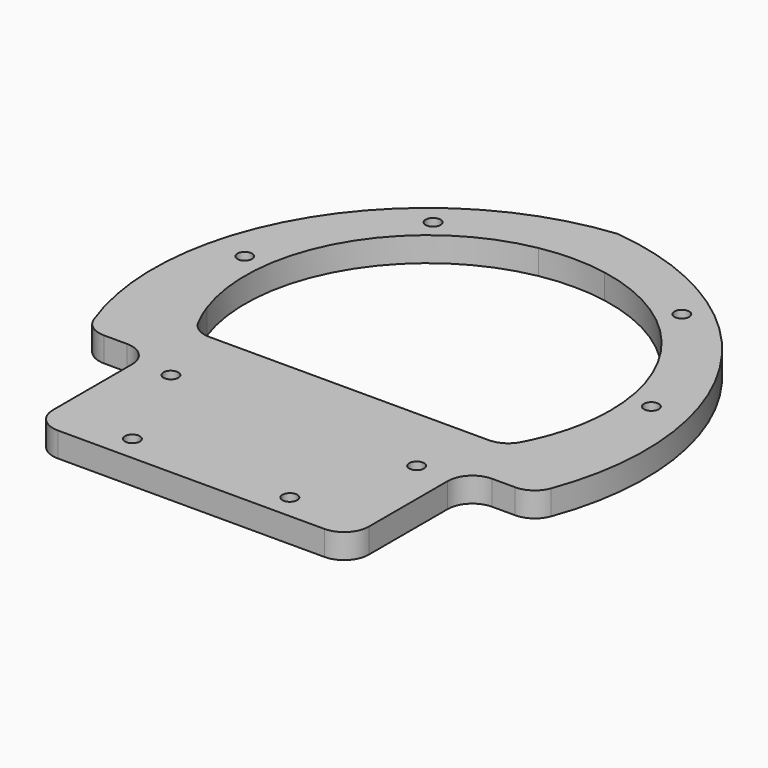
from build123d import *

# Parameters (mm, degrees)
F0_R     = 1.5
F1_DEPTH = 5
F2_R     = 5


# Not quite as in the source:
# - a feature names something its author has since deleted; it is built from what else it names


with BuildPart() as f1:
    # F0 (on Top) → F1 (new body)
    with BuildSketch(Plane.XY):
        with BuildLine():
            Line((32, -25.9806431703), (45.0002060157, -25.9806431703))
            Line((45.0002060157, -25.9806431703), (34.8648160141, -8.425632733))
            ThreePointArc((34.8648160141, -8.425632733), (33.2306953855, -12.3086021935), (31.1657699329, -15.9806431703))
            Line((31.1657699329, -15.9806431703), (32, -15.9806431703))
            Line((32, -15.9806431703), (32, -25.9806431703))
        make_face()
        with BuildLine():
            Line((34.8648160141, -8.425632733), (45.0002060157, -25.9806431703))
            ThreePointArc((45.0002060157, -25.9806431703), (42.4187903028, 24.4905), (0.0002060157, 51.9616431703))
            Line((0.0002060157, 51.9616431703), (6.7047123911, 40.3490974884))
            ThreePointArc((6.7047123911, 40.3490974884), (28.4347881869, 27.6357391565), (37, 3.9616431703))
            ThreePointArc((37, 3.9616431703), (36.4622969142, -2.3233312719), (34.8648160141, -8.425632733))
        make_face()
        with Locations((41.2026322213, 9.0961922878)):
            Circle(F0_R, mode=Mode.SUBTRACT)
        with Locations((25.2027902051, 36.8090964203)):
            Circle(F0_R, mode=Mode.SUBTRACT)
        with BuildLine():
            Line((32, -55.9806431703), (32, -25.9806431703))
            Line((32, -25.9806431703), (21.7361332508, -25.9806431703))
            ThreePointArc((21.7361332508, -25.9806431703), (0, -33.0383568297), (-21.7361332508, -25.9806431703))
            Line((-21.7361332508, -25.9806431703), (-32, -25.9806431703))
            Line((-32, -25.9806431703), (-32, -55.9806431703))
            Line((-32, -55.9806431703), (32, -55.9806431703))
        make_face()
        with Locations((-16, -50.8592247836)):
            Circle(F0_R, mode=Mode.SUBTRACT)
        with Locations((-24.9, -29.9806431703)):
            Circle(F0_R, mode=Mode.SUBTRACT)
        with Locations((16, -50.9806431703)):
            Circle(F0_R, mode=Mode.SUBTRACT)
        with Locations((24.9, -29.9806431703)):
            Circle(F0_R, mode=Mode.SUBTRACT)
        with BuildLine():
            Line((21.7361332508, -25.9806431703), (32, -25.9806431703))
            Line((32, -25.9806431703), (32, -15.9806431703))
            Line((32, -15.9806431703), (31.1657699329, -15.9806431703))
            ThreePointArc((31.1657699329, -15.9806431703), (26.9193766665, -21.422350997), (21.7361332508, -25.9806431703))
        make_face()
        with BuildLine():
            Line((6.7047123911, 40.3490974884), (0.0002060157, 51.9616431703))
            Line((0.0002060157, 51.9616431703), (-6.7042513108, 40.3491824435))
            ThreePointArc((-6.7042513108, 40.3491824435), (0.0002344208, 40.9616431696), (6.7047123911, 40.3490974884))
        make_face()
        with BuildLine():
            Line((-6.7042513108, 40.3491824435), (0.0002060157, 51.9616431703))
            ThreePointArc((0.0002060157, 51.9616431703), (-42.4183782713, 24.4905), (-44.9997939843, -25.9806431703))
            Line((-44.9997939843, -25.9806431703), (-34.8646590472, -8.4260745178))
            ThreePointArc((-34.8646590472, -8.4260745178), (-32.04293994, 22.4616431703), (-6.7042513108, 40.3491824435))
        make_face()
        with Locations((-41.202520651, 9.0964271731)):
            Circle(F0_R, mode=Mode.SUBTRACT)
        with Locations((-25.202520651, 36.8092400942)):
            Circle(F0_R, mode=Mode.SUBTRACT)
        with BuildLine():
            ThreePointArc((-21.7361332508, -25.9806431703), (0, -33.0383568297), (21.7361332508, -25.9806431703))
            Line((21.7361332508, -25.9806431703), (-21.7361332508, -25.9806431703))
        make_face()
        with BuildLine():
            Line((-21.7361332508, -25.9806431703), (21.7361332508, -25.9806431703))
            ThreePointArc((21.7361332508, -25.9806431703), (26.9193766665, -21.422350997), (31.1657699329, -15.9806431703))
            Line((31.1657699329, -15.9806431703), (-31.1657699329, -15.9806431703))
            ThreePointArc((-31.1657699329, -15.9806431703), (-26.9193766665, -21.422350997), (-21.7361332508, -25.9806431703))
        make_face()
        with BuildLine():
            Line((-34.8646590472, -8.4260745178), (-44.9997939843, -25.9806431703))
            Line((-44.9997939843, -25.9806431703), (-32, -25.9806431703))
            Line((-32, -25.9806431703), (-32, -15.9806431703))
            Line((-32, -15.9806431703), (-31.1657699329, -15.9806431703))
            ThreePointArc((-31.1657699329, -15.9806431703), (-33.2305923015, -12.3088127328), (-34.8646590472, -8.4260745178))
        make_face()
        with BuildLine():
            Line((-32, -25.9806431703), (-21.7361332508, -25.9806431703))
            ThreePointArc((-21.7361332508, -25.9806431703), (-26.9193766665, -21.422350997), (-31.1657699329, -15.9806431703))
            Line((-31.1657699329, -15.9806431703), (-32, -15.9806431703))
            Line((-32, -15.9806431703), (-32, -25.9806431703))
        make_face()
    extrude(amount=F1_DEPTH)

    # F2
    f2_edges = [f1.edges().sort_by_distance(p)[0] for p in [
        (-32, -25.980643, 2.5),
        (-44.999794, -25.980643, 2.5),
        (32, -25.980643, 2.5),
        (45.000206, -25.980643, 2.5),
        (-32, -55.980643, 2.5),
        (32, -55.980643, 2.5),
        (-31.16577, -15.980643, 2.5),
        (31.16577, -15.980643, 2.5),
    ]]
    fillet(f2_edges, radius=F2_R)


solid = f1.part
